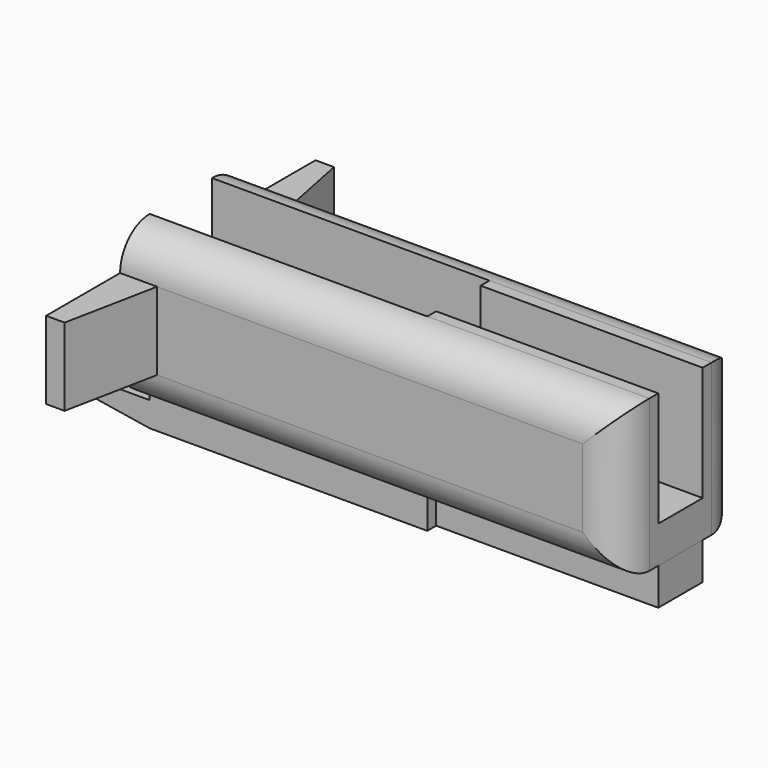
from build123d import *

# Parameters (mm, degrees)
F0_W         = 12
F0_H         = 3
F1_DEPTH     = 2
F2_DEPTH     = 8.2
F3_R         = 2
F4_DEPTH     = 2
F5_W         = 4.2
F5_H         = 1.34
F6_DEPTH     = 5
F7_W         = 4.2
F7_H         = 1.34
F8_DEPTH     = 5
F9_SIZE2     = 5
F9_SIZE      = 0.8
F9_2_SIZE2   = 5
F9_2_SIZE    = 0.8
F11_W        = 2
F11_H        = 4.2
F12_DEPTH    = 5
F10_W        = 2
F10_H        = 4.2
F13_DEPTH    = 5
F14_T4_DEPTH = 30.181320863
F14_T9_DEPTH = 30.181320863


# Not quite as in the source:
# - a fillet or chamfer that OpenCascade refuses, or shapes differently, is made with other operations: its cross-section is extruded or revolved along the edge and cut away or added
# - two fillets or chamfers of one size are made in one step


with BuildPart() as f1:
    # F0 (on Top) → F1 (new body)
    with BuildSketch(Plane.XY):
        Polygon((7.5, 1.5), (7.5, 2.1), (-7.5, 2.1), (-7.5, -2.1), (7.5, -2.1), (7.5, -1.5), align=None)
        with Locations((13.5, 0)):
            Rectangle(F0_W, F0_H)
        Polygon((-7.5, 2.1), (7.5, 2.1), (7.5, 1.5), (19.5, 1.5), (19.5, 4.1), (-7.5, 4.1), align=None)
        Polygon((7.5, -2.1), (-7.5, -2.1), (-7.5, -4.1), (19.5, -4.1), (19.5, -1.5), (7.5, -1.5), align=None)
    extrude(amount=F1_DEPTH)

    # F0 (on Top) → F2 (join)
    with BuildSketch(Plane.XY):
        Polygon((7.5, -2.1), (-7.5, -2.1), (-7.5, -4.1), (19.5, -4.1), (19.5, -1.5), (7.5, -1.5), align=None)
        Polygon((-7.5, 2.1), (7.5, 2.1), (7.5, 1.5), (19.5, 1.5), (19.5, 4.1), (-7.5, 4.1), align=None)
    extrude(amount=F2_DEPTH)

    # F3
    f3_edges = [f1.edges().sort_by_distance(p)[0] for p in [
        (19.5, -4.1, 4.1),
        (19.5, 4.1, 4.1),
        (6, -4.1, 8.2),
        (6, 4.1, 8.2),
        (6, 4.1, 0),
        (6, -4.1, 0),
    ]]
    fillet(f3_edges, radius=F3_R)

    # F7 (on face) → F8 (join)
    with BuildSketch(Plane(origin=(-7.5, 0, 0), x_dir=(0, -1, 0), z_dir=(-1, 0, 0))):
        with Locations((0, 0.67)):
            Rectangle(F7_W, F7_H)
    extrude(amount=F8_DEPTH)

    # F9#2
    f9_2_edges = [f1.edges().sort_by_distance(p)[0] for p in [
        (-12.5, 0, 0),
    ]]
    f9_2_side = f1.faces().sort_by_distance((-12.5, 0, 0.67))[0]
    chamfer(f9_2_edges, length=F9_2_SIZE, length2=F9_2_SIZE2, reference=f9_2_side)

    # F11 (on face) → F12 (join)
    with BuildSketch(Plane(origin=(0, 4.1, 0), x_dir=(-1, 0, 0), z_dir=(0, 1, 0))):
        with Locations((6.5, 4.1)):
            Rectangle(F11_W, F11_H)
    extrude(amount=F12_DEPTH)

    # F10 (on face) → F13 (join)
    with BuildSketch(Plane.XZ.offset(4.1)):
        with Locations((-6.5, 4.1)):
            Rectangle(F10_W, F10_H)
    extrude(amount=F13_DEPTH)

    # F14: chamfer of 1 x 5 on 2 edges, made by hand


with BuildPart() as f4:
    # F0 (on Top) → F4 (new body)
    with BuildSketch(Plane.XY):
        with Locations((13.5, 0)):
            Rectangle(F0_W, F0_H)
        Polygon((7.5, 1.5), (7.5, 2.1), (-7.5, 2.1), (-7.5, -2.1), (7.5, -2.1), (7.5, -1.5), align=None)
    extrude(amount=-F4_DEPTH)

    # F5 (on face) → F6 (join)
    with BuildSketch(Plane(origin=(-7.5, 0, 0), x_dir=(0, -1, 0), z_dir=(-1, 0, 0))):
        with Locations((0, -1.33)):
            Rectangle(F5_W, F5_H)
    extrude(amount=F6_DEPTH)

    # F9
    f9_edges = [f4.edges().sort_by_distance(p)[0] for p in [
        (-12.5, 0, -2),
    ]]
    f9_side = f4.faces().sort_by_distance((-12.5, 0, -1.33))[0]
    chamfer(f9_edges, length=F9_SIZE, length2=F9_SIZE2, reference=f9_side)


with BuildPart() as f14_tool2:
    # F14_s3 → F14_t4 (new body)
    with BuildSketch(Plane.XY.offset(-10.9906604315)):
        Polygon((-6.5, -9.1), (-5.5, -4.1), (-5.5, -9.1), align=None)
    extrude(amount=F14_T4_DEPTH)

    split(bisect_by=Plane.XZ.offset(4.1), keep=Keep.TOP)


with BuildPart() as f1_1:
    add(f1.part)

    # F14_t1: cut F14_tool2
    add(f14_tool2.part, mode=Mode.SUBTRACT)


with BuildPart() as f14_tool7:
    # F14_s8 → F14_t9 (new body)
    with BuildSketch(Plane.XY.offset(19.1906604315)):
        Polygon((-6.5, 9.1), (-5.5, 4.1), (-5.5, 9.1), align=None)
    extrude(amount=-F14_T9_DEPTH)

    split(bisect_by=Plane.XZ.offset(-4.1), keep=Keep.BOTTOM)


with BuildPart() as f1_2:
    add(f1_1.part)

    # F14_t6: cut F14_tool7
    add(f14_tool7.part, mode=Mode.SUBTRACT)


solid = Compound([f4.part, f1_2.part])
